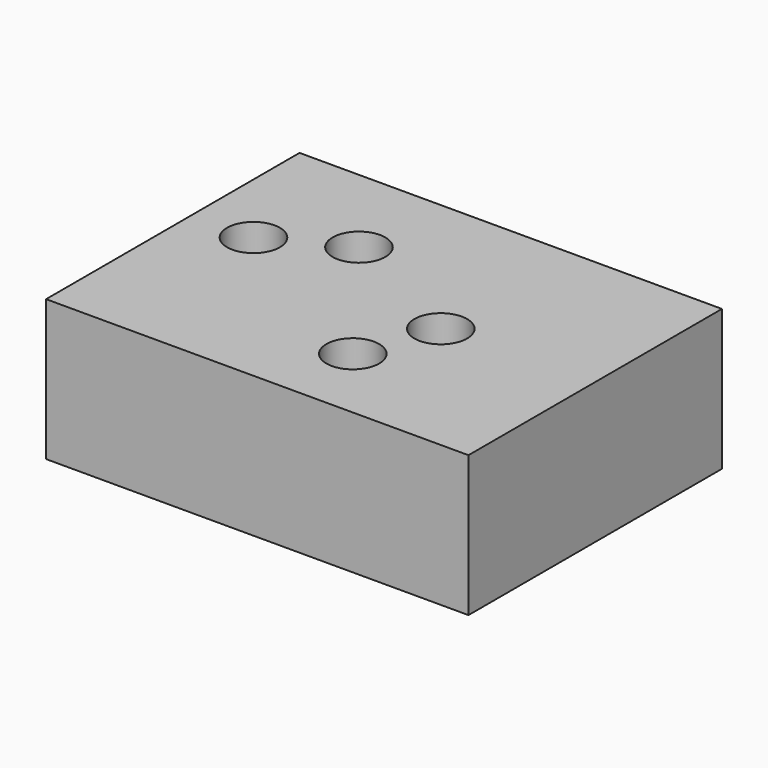
from build123d import *

# Parameters (mm, degrees)
F0_W     = 76.2
F0_H     = 57.15
F1_DEPTH = 25.4
F3_D     = 9.525


# Not quite as in the source:
# - a length typed as a fraction of an inch, garbled in the dataset ("3 / 203.2 mm" for 3/8 in), is restored


with BuildPart() as f1:
    # F0 (on Top) → F1 (new body)
    with BuildSketch(Plane.XY):
        with Locations((38.1, -28.575)):
            Rectangle(F0_W, F0_H)
    extrude(amount=F1_DEPTH)

    # F3 (through all)
    with Locations(Plane.XY.offset(25.4)):
        with Locations((49.0540005267, -29.4691771269), (24.5114304125, -17.2301307321), (11.0678356141, -24.2150630802), (44.1506654024, -43.1743003428)):
            Hole(F3_D / 2)


solid = f1.part
